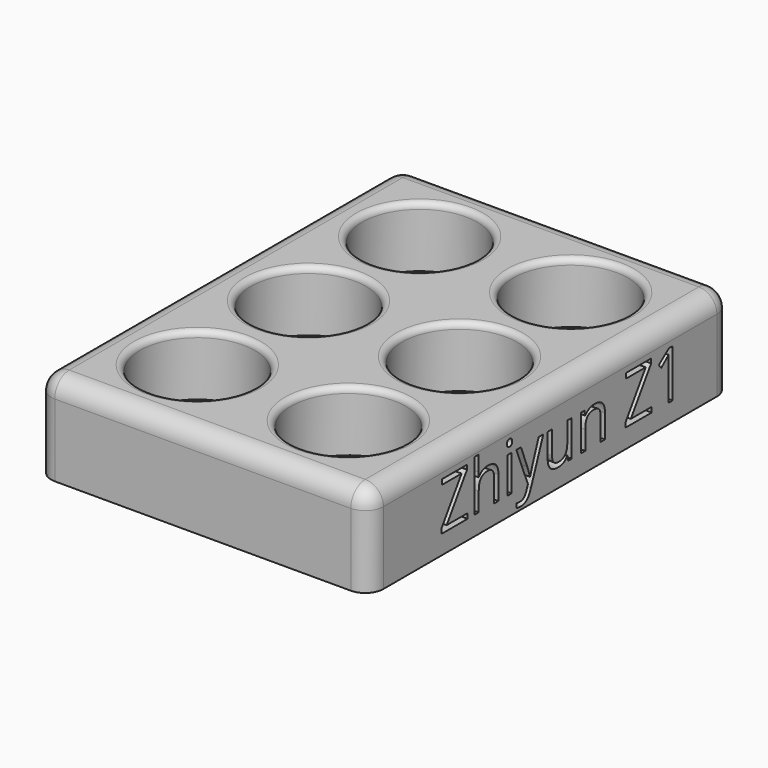
from build123d import *

# Parameters (mm, degrees)
F0_W         = 55
F0_H         = 75
F0_R         = 9.5
F1_DEPTH     = 15
F2_DEPTH     = 5
F3_R         = 3
F4_TEXT_SIZE = 11.1111111111
F5_DEPTH     = 2
F6_R         = 1


# Not quite as in the source:
# - Text() gives the source's letters only with a copy of the font that has no kerning and outlines rounded to 1/6400 em; it was checked with that copy


with BuildPart() as f1:
    # F0 (on Top) → F1 (new body)
    with BuildSketch(Plane.XY):
        Rectangle(F0_W, F0_H)
        with Locations((-12.5, -23)):
            Circle(F0_R, mode=Mode.SUBTRACT)
        with Locations((12.5, -23)):
            Circle(F0_R, mode=Mode.SUBTRACT)
        with Locations((-12.5, 0)):
            Circle(F0_R, mode=Mode.SUBTRACT)
        with Locations((-12.5, 23)):
            Circle(F0_R, mode=Mode.SUBTRACT)
        with Locations((12.5, 0)):
            Circle(F0_R, mode=Mode.SUBTRACT)
        with Locations((12.5, 23)):
            Circle(F0_R, mode=Mode.SUBTRACT)
    extrude(amount=F1_DEPTH)

    # F0 (on Top) → F2 (join)
    with BuildSketch(Plane.XY):
        with Locations((12.5, -23)):
            Circle(F0_R)
        with Locations((12.5, 0)):
            Circle(F0_R)
        with Locations((12.5, 23)):
            Circle(F0_R)
        with Locations((-12.5, 23)):
            Circle(F0_R)
        with Locations((-12.5, -23)):
            Circle(F0_R)
        with Locations((-12.5, 0)):
            Circle(F0_R)
    extrude(amount=F2_DEPTH)

    # F3
    f3_edges = [f1.edges().sort_by_distance(p)[0] for p in [
        (27.5, -37.5, 7.5),
        (27.5, 0, 15),
        (0, -37.5, 15),
        (-27.5, -37.5, 7.5),
        (-27.5, 0, 15),
        (0, 37.5, 15),
        (27.5, 37.5, 7.5),
        (-27.5, 37.5, 7.5),
    ]]
    fillet(f3_edges, radius=F3_R)

    # F4 (on face) → F5 (cut)
    with BuildSketch(Plane.YZ.offset(27.5)):
        with Locations((-22.973129815, 3.1474459912)):
            Text('Zhiyun Z1', F4_TEXT_SIZE, font='Open Sans', text_align=(TextAlign.LEFT, TextAlign.BOTTOM))
    extrude(amount=-F5_DEPTH, mode=Mode.SUBTRACT)

    # F6
    f6_edges = [f1.edges().sort_by_distance(p)[0] for p in [
        (3, -23, 15),
        (-22, -23, 15),
        (-22, 0, 15),
        (3, 0, 15),
        (-22, 23, 15),
        (3, 23, 15),
    ]]
    fillet(f6_edges, radius=F6_R)


solid = f1.part
